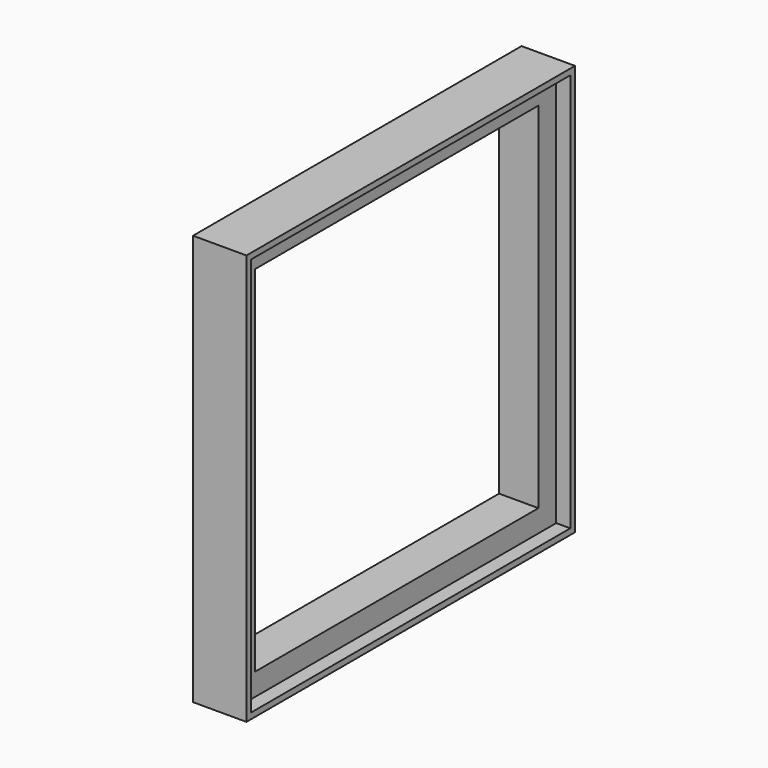
from build123d import *

# Parameters (mm, degrees)
F0_W     = 146
F0_H     = 146
F1_DEPTH = 19
F2_W     = 126
F2_H     = 126
F3_DEPTH = 25
F4_W     = 141.8
F4_H     = 141.8
F5_DEPTH = 5


# Not quite as in the source:
# - a feature names something its author has since deleted; it is built from what else it names


with BuildPart() as f1:
    # F0 (on Right) → F1 (new body)
    with BuildSketch(Plane.YZ):
        with Locations((17.8558837175, 26.935071826)):
            Rectangle(F0_W, F0_H)
    extrude(amount=F1_DEPTH)

    # F2 (on face) → F3 (cut)
    with BuildSketch(Plane.YZ.offset(19)):
        with Locations((17.8558837175, 26.935071826)):
            Rectangle(F2_W, F2_H)
    extrude(amount=-F3_DEPTH, mode=Mode.SUBTRACT)

    # F4 (on face) → F5 (cut)
    with BuildSketch(Plane.YZ.offset(19)):
        with Locations((17.8558837175, 26.935071826)):
            Rectangle(F4_W, F4_H)
    extrude(amount=-F5_DEPTH, mode=Mode.SUBTRACT)


solid = f1.part
